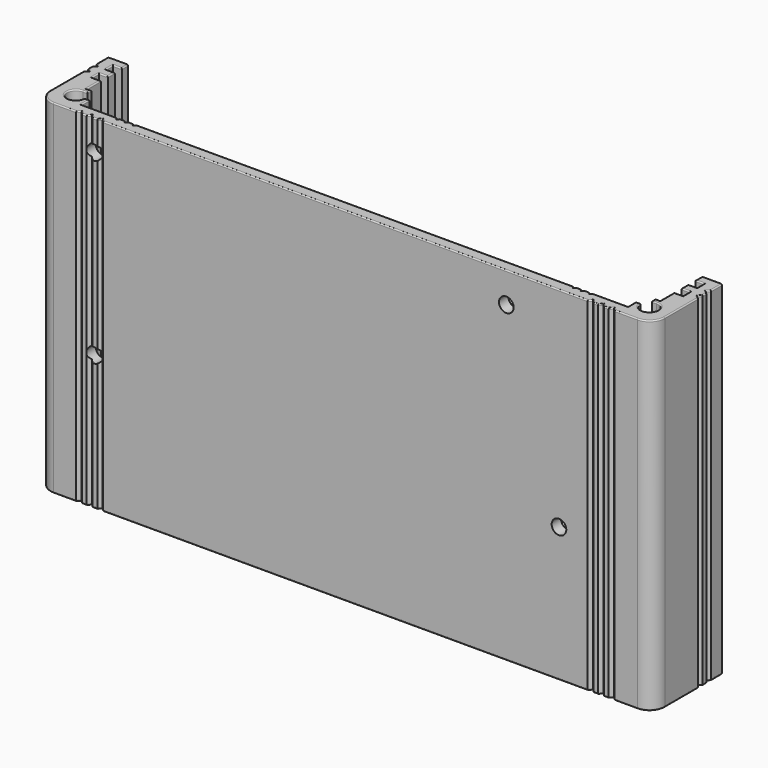
from build123d import *

# Parameters (mm, degrees)
F1_DEPTH     = 58.7
F2_R         = 0.2
F3_R         = 0.2
F4_T1_DEPTH  = 58.7
F4_T4_ANGLE  = 90
F4_T6_ANGLE  = 90
F4_T8_ANGLE  = 90
F4_T10_ANGLE = 90
F4_T12_ANGLE = 90
F4_T14_ANGLE = 90
F4_T16_ANGLE = 90
F4_T18_ANGLE = 90
F5_T1_DEPTH  = 58.7
F5_T4_ANGLE  = 90
F5_T6_ANGLE  = 90
F5_T8_ANGLE  = 90
F5_T10_ANGLE = 90
F6_R         = 1.25
F7_DEPTH     = 2


# Not quite as in the source:
# - a fillet or chamfer that OpenCascade refuses, or shapes differently, is made with other operations: its cross-section is extruded or revolved along the edge and cut away or added


with BuildPart() as f1:
    # F0 (on Top) → F1 (new body)
    with BuildSketch(Plane.XY):
        with BuildLine():
            Line((-52.5, -5.3), (-52.5, -15))
            Line((-52.5, -15), (-46, -15))
            Line((-46, -15), (-45.5, -14.5))
            Line((-45.5, -14.5), (-45, -15))
            Line((-45, -15), (-44.2, -15))
            Line((-44.2, -15), (-43.7, -14.5))
            Line((-43.7, -14.5), (-43.2, -15))
            Line((-43.2, -15), (-42.4, -15))
            Line((-42.4, -15), (-41.9, -14.5))
            Line((-41.9, -14.5), (-41.4, -15))
            Line((-41.4, -15), (0, -15))
            Line((0, -15), (41.4, -15))
            Line((41.4, -15), (41.9, -14.5))
            Line((41.9, -14.5), (42.4, -15))
            Line((42.4, -15), (43.2, -15))
            Line((43.2, -15), (43.7, -14.5))
            Line((43.7, -14.5), (44.2, -15))
            Line((44.2, -15), (45, -15))
            Line((45, -15), (45.5, -14.5))
            Line((45.5, -14.5), (46, -15))
            Line((46, -15), (52.5, -15))
            Line((52.5, -15), (52.5, -5.3))
            Line((52.5, -5.3), (52, -4.8))
            Line((52, -4.8), (52.5, -4.3))
            Line((52.5, -4.3), (52.5, -3.5))
            Line((52.5, -3.5), (52, -3))
            Line((52, -3), (52.5, -2.5))
            Line((52.5, -2.5), (52.5, 0))
            Line((52.5, 0), (49, 0))
            Line((49, 0), (49, -1.5))
            Line((49, -1.5), (50.5, -1.5))
            Line((50.5, -1.5), (50.5, -3))
            Line((50.5, -3), (49, -3))
            Line((49, -3), (49, -4.5))
            Line((49, -4.5), (50.5, -4.5))
            Line((50.5, -4.5), (50.5, -6))
            Line((50.5, -6), (49, -6))
            Line((49, -6), (49, -9))
            Line((49, -9), (48.2, -9))
            Line((48.2, -9), (48.2, -9.8))
            Line((48.2, -9.8), (49, -9.8))
            ThreePointArc((49, -9.8), (50.0606601718, -12.3606601718), (47.5, -11.3))
            Line((47.5, -11.3), (46.7, -11.3))
            Line((46.7, -11.3), (46.7, -13))
            Line((46.7, -13), (40.7, -13))
            Line((40.7, -13), (40.4, -13.3))
            Line((40.4, -13.3), (40.1, -13))
            Line((40.1, -13), (39.3, -13))
            Line((39.3, -13), (39, -13.3))
            Line((39, -13.3), (38.7, -13))
            Line((38.7, -13), (37.9, -13))
            Line((37.9, -13), (37.6, -13.3))
            Line((37.6, -13.3), (37.3, -13))
            Line((37.3, -13), (0, -13))
            Line((0, -13), (-37.3, -13))
            Line((-37.3, -13), (-37.6, -13.3))
            Line((-37.6, -13.3), (-37.9, -13))
            Line((-37.9, -13), (-38.7, -13))
            Line((-38.7, -13), (-39, -13.3))
            Line((-39, -13.3), (-39.3, -13))
            Line((-39.3, -13), (-40.1, -13))
            Line((-40.1, -13), (-40.4, -13.3))
            Line((-40.4, -13.3), (-40.7, -13))
            Line((-40.7, -13), (-46.7, -13))
            Line((-46.7, -13), (-46.7, -11.3))
            Line((-46.7, -11.3), (-47.5, -11.3))
            ThreePointArc((-47.5, -11.3), (-50.0606601718, -12.3606601718), (-49, -9.8))
            Line((-49, -9.8), (-48.2, -9.8))
            Line((-48.2, -9.8), (-48.2, -9))
            Line((-48.2, -9), (-49, -9))
            Line((-49, -9), (-49, -6))
            Line((-49, -6), (-50.5, -6))
            Line((-50.5, -6), (-50.5, -4.5))
            Line((-50.5, -4.5), (-49, -4.5))
            Line((-49, -4.5), (-49, -3))
            Line((-49, -3), (-50.5, -3))
            Line((-50.5, -3), (-50.5, -1.5))
            Line((-50.5, -1.5), (-49, -1.5))
            Line((-49, -1.5), (-49, 0))
            Line((-49, 0), (-52.5, 0))
            Line((-52.5, 0), (-52.5, -2.5))
            Line((-52.5, -2.5), (-52, -3))
            Line((-52, -3), (-52.5, -3.5))
            Line((-52.5, -3.5), (-52.5, -4.3))
            Line((-52.5, -4.3), (-52, -4.8))
            Line((-52, -4.8), (-52.5, -5.3))
        make_face()
    extrude(amount=F1_DEPTH)

    # F2
    f2_edges = [f1.edges().sort_by_distance(p)[0] for p in [
        (-52.5, -10.15, 58.7),
        (-49.25, -15, 58.7),
        (-45.75, -14.75, 58.7),
        (-45.25, -14.75, 58.7),
        (-44.6, -15, 58.7),
        (-43.95, -14.75, 58.7),
        (-43.45, -14.75, 58.7),
        (-42.8, -15, 58.7),
        (-42.15, -14.75, 58.7),
        (-41.65, -14.75, 58.7),
        (0, -15, 58.7),
        (41.65, -14.75, 58.7),
        (42.15, -14.75, 58.7),
        (42.8, -15, 58.7),
        (43.45, -14.75, 58.7),
        (43.95, -14.75, 58.7),
        (44.6, -15, 58.7),
        (45.25, -14.75, 58.7),
        (45.75, -14.75, 58.7),
        (49.25, -15, 58.7),
        (52.5, -10.15, 58.7),
        (52.25, -5.05, 58.7),
        (52.25, -4.55, 58.7),
        (52.5, -3.9, 58.7),
        (52.25, -3.25, 58.7),
        (52.25, -2.75, 58.7),
        (52.5, -1.25, 58.7),
        (50.75, 0, 58.7),
        (49, -0.75, 58.7),
        (49.75, -1.5, 58.7),
        (50.5, -2.25, 58.7),
        (49.75, -3, 58.7),
        (49, -3.75, 58.7),
        (49.75, -4.5, 58.7),
        (50.5, -5.25, 58.7),
        (49.75, -6, 58.7),
        (49, -7.5, 58.7),
        (48.6, -9, 58.7),
        (48.2, -9.4, 58.7),
        (48.6, -9.8, 58.7),
        (50.06066, -12.36066, 58.7),
        (47.1, -11.3, 58.7),
        (46.7, -12.15, 58.7),
        (43.7, -13, 58.7),
        (40.55, -13.15, 58.7),
        (40.25, -13.15, 58.7),
        (39.7, -13, 58.7),
        (39.15, -13.15, 58.7),
        (38.85, -13.15, 58.7),
        (38.3, -13, 58.7),
        (37.75, -13.15, 58.7),
        (37.45, -13.15, 58.7),
        (0, -13, 58.7),
        (-37.45, -13.15, 58.7),
        (-37.75, -13.15, 58.7),
        (-38.3, -13, 58.7),
        (-38.85, -13.15, 58.7),
        (-39.15, -13.15, 58.7),
        (-39.7, -13, 58.7),
        (-40.25, -13.15, 58.7),
        (-40.55, -13.15, 58.7),
        (-43.7, -13, 58.7),
        (-46.7, -12.15, 58.7),
        (-47.1, -11.3, 58.7),
        (-50.06066, -12.36066, 58.7),
        (-48.6, -9.8, 58.7),
        (-48.2, -9.4, 58.7),
        (-48.6, -9, 58.7),
        (-49, -7.5, 58.7),
        (-49.75, -6, 58.7),
        (-50.5, -5.25, 58.7),
        (-49.75, -4.5, 58.7),
        (-49, -3.75, 58.7),
        (-49.75, -3, 58.7),
        (-50.5, -2.25, 58.7),
        (-49.75, -1.5, 58.7),
        (-49, -0.75, 58.7),
        (-50.75, 0, 58.7),
        (-52.5, -1.25, 58.7),
        (-52.25, -2.75, 58.7),
        (-52.25, -3.25, 58.7),
        (-52.5, -3.9, 58.7),
        (-52.25, -4.55, 58.7),
        (-52.25, -5.05, 58.7),
    ]]
    fillet(f2_edges, radius=F2_R)

    # F3
    f3_edges = [f1.edges().sort_by_distance(p)[0] for p in [
        (-52.5, -10.15, 0),
        (-49.25, -15, 0),
        (-45.75, -14.75, 0),
        (-45.25, -14.75, 0),
        (-44.6, -15, 0),
        (-43.95, -14.75, 0),
        (-43.45, -14.75, 0),
        (-42.8, -15, 0),
        (-42.15, -14.75, 0),
        (-41.65, -14.75, 0),
        (0, -15, 0),
        (41.65, -14.75, 0),
        (42.15, -14.75, 0),
        (42.8, -15, 0),
        (43.45, -14.75, 0),
        (43.95, -14.75, 0),
        (44.6, -15, 0),
        (45.25, -14.75, 0),
        (45.75, -14.75, 0),
        (49.25, -15, 0),
        (52.5, -10.15, 0),
        (52.25, -5.05, 0),
        (52.25, -4.55, 0),
        (52.5, -3.9, 0),
        (52.25, -3.25, 0),
        (52.25, -2.75, 0),
        (52.5, -1.25, 0),
        (50.75, 0, 0),
        (49, -0.75, 0),
        (49.75, -1.5, 0),
        (50.5, -2.25, 0),
        (49.75, -3, 0),
        (49, -3.75, 0),
        (49.75, -4.5, 0),
        (50.5, -5.25, 0),
        (49.75, -6, 0),
        (49, -7.5, 0),
        (48.6, -9, 0),
        (48.2, -9.4, 0),
        (48.6, -9.8, 0),
        (50.06066, -12.36066, 0),
        (47.1, -11.3, 0),
        (46.7, -12.15, 0),
        (43.7, -13, 0),
        (40.55, -13.15, 0),
        (40.25, -13.15, 0),
        (39.7, -13, 0),
        (39.15, -13.15, 0),
        (38.85, -13.15, 0),
        (38.3, -13, 0),
        (37.75, -13.15, 0),
        (37.45, -13.15, 0),
        (0, -13, 0),
        (-37.45, -13.15, 0),
        (-37.75, -13.15, 0),
        (-38.3, -13, 0),
        (-38.85, -13.15, 0),
        (-39.15, -13.15, 0),
        (-39.7, -13, 0),
        (-40.25, -13.15, 0),
        (-40.55, -13.15, 0),
        (-43.7, -13, 0),
        (-46.7, -12.15, 0),
        (-47.1, -11.3, 0),
        (-50.06066, -12.36066, 0),
        (-48.6, -9.8, 0),
        (-48.2, -9.4, 0),
        (-48.6, -9, 0),
        (-49, -7.5, 0),
        (-49.75, -6, 0),
        (-50.5, -5.25, 0),
        (-49.75, -4.5, 0),
        (-49, -3.75, 0),
        (-49.75, -3, 0),
        (-50.5, -2.25, 0),
        (-49.75, -1.5, 0),
        (-49, -0.75, 0),
        (-50.75, 0, 0),
        (-52.5, -1.25, 0),
        (-52.25, -2.75, 0),
        (-52.25, -3.25, 0),
        (-52.5, -3.9, 0),
        (-52.25, -4.55, 0),
        (-52.25, -5.05, 0),
    ]]
    fillet(f3_edges, radius=F3_R)

    # F4: fillet of radius 0.3 on 4 edges, made by hand

    # F4_s2 → F4_t1 (cut)
    with BuildSketch(Plane.XY):
        with BuildLine():
            ThreePointArc((-52.5, -0.3), (-52.4121320344, -0.0878679656), (-52.2, 0))
            Line((-52.2, 0), (-52.5, 0))
            Line((-52.5, 0), (-52.5, -0.3))
        make_face()
        with BuildLine():
            ThreePointArc((-49.3, 0), (-49.0878679656, -0.0878679656), (-49, -0.3))
            Line((-49, -0.3), (-49, 0))
            Line((-49, 0), (-49.3, 0))
        make_face()
        with BuildLine():
            ThreePointArc((49.3, 0), (49.0878679656, -0.0878679656), (49, -0.3))
            Line((49, -0.3), (49, 0))
            Line((49, 0), (49.3, 0))
        make_face()
        with BuildLine():
            ThreePointArc((52.5, -0.3), (52.4121320344, -0.0878679656), (52.2, 0))
            Line((52.2, 0), (52.5, 0))
            Line((52.5, 0), (52.5, -0.3))
        make_face()
    extrude(amount=F4_T1_DEPTH, mode=Mode.SUBTRACT)

    # F4_s3 → F4_t4 (revolve, cut)
    with BuildSketch(Plane.YZ.offset(52.2)):
        with BuildLine():
            ThreePointArc((-0.2, 0), (-0.0585786438, 0.0585786438), (0, 0.2))
            Line((0, 0.2), (0, 0))
            Line((0, 0), (-0.2, 0))
        make_face()
    revolve(axis=Axis((52.2, -0.3, 0), (0, 0, -1)), revolution_arc=F4_T4_ANGLE, mode=Mode.SUBTRACT)

    # F4_s5 → F4_t6 (revolve, cut)
    with BuildSketch(Plane.XZ.offset(0.3)):
        with BuildLine():
            ThreePointArc((52.3, 58.7), (52.4414213562, 58.6414213562), (52.5, 58.5))
            Line((52.5, 58.5), (52.5, 58.7))
            Line((52.5, 58.7), (52.3, 58.7))
        make_face()
    revolve(axis=Axis((52.2, -0.3, 58.7), (0, 0, 1)), revolution_arc=F4_T6_ANGLE, mode=Mode.SUBTRACT)

    # F4_s7 → F4_t8 (revolve, cut)
    with BuildSketch(Plane.XZ.offset(0.3)):
        with BuildLine():
            ThreePointArc((49.2, 0), (49.0585786438, 0.0585786438), (49, 0.2))
            Line((49, 0.2), (49, 0))
            Line((49, 0), (49.2, 0))
        make_face()
    revolve(axis=Axis((49.3, -0.3, 0), (0, 0, -1)), revolution_arc=F4_T8_ANGLE, mode=Mode.SUBTRACT)

    # F4_s9 → F4_t10 (revolve, cut)
    with BuildSketch(Plane.YZ.offset(49.3)):
        with BuildLine():
            ThreePointArc((-0.2, 58.7), (-0.0585786438, 58.6414213562), (0, 58.5))
            Line((0, 58.5), (0, 58.7))
            Line((0, 58.7), (-0.2, 58.7))
        make_face()
    revolve(axis=Axis((49.3, -0.3, 58.7), (0, 0, 1)), revolution_arc=F4_T10_ANGLE, mode=Mode.SUBTRACT)

    # F4_s11 → F4_t12 (revolve, cut)
    with BuildSketch(Plane.YZ.offset(-49.3)):
        with BuildLine():
            ThreePointArc((-0.2, 0), (-0.0585786438, 0.0585786438), (0, 0.2))
            Line((0, 0.2), (0, 0))
            Line((0, 0), (-0.2, 0))
        make_face()
    revolve(axis=Axis((-49.3, -0.3, 0), (0, 0, -1)), revolution_arc=F4_T12_ANGLE, mode=Mode.SUBTRACT)

    # F4_s13 → F4_t14 (revolve, cut)
    with BuildSketch(Plane.XZ.offset(0.3)):
        with BuildLine():
            ThreePointArc((-49.2, 58.7), (-49.0585786438, 58.6414213562), (-49, 58.5))
            Line((-49, 58.5), (-49, 58.7))
            Line((-49, 58.7), (-49.2, 58.7))
        make_face()
    revolve(axis=Axis((-49.3, -0.3, 58.7), (0, 0, 1)), revolution_arc=F4_T14_ANGLE, mode=Mode.SUBTRACT)

    # F4_s15 → F4_t16 (revolve, cut)
    with BuildSketch(Plane.XZ.offset(0.3)):
        with BuildLine():
            ThreePointArc((-52.3, 0), (-52.4414213562, 0.0585786438), (-52.5, 0.2))
            Line((-52.5, 0.2), (-52.5, 0))
            Line((-52.5, 0), (-52.3, 0))
        make_face()
    revolve(axis=Axis((-52.2, -0.3, 0), (0, 0, -1)), revolution_arc=F4_T16_ANGLE, mode=Mode.SUBTRACT)

    # F4_s17 → F4_t18 (revolve, cut)
    with BuildSketch(Plane.YZ.offset(-52.2)):
        with BuildLine():
            ThreePointArc((-0.2, 58.7), (-0.0585786438, 58.6414213562), (0, 58.5))
            Line((0, 58.5), (0, 58.7))
            Line((0, 58.7), (-0.2, 58.7))
        make_face()
    revolve(axis=Axis((-52.2, -0.3, 58.7), (0, 0, 1)), revolution_arc=F4_T18_ANGLE, mode=Mode.SUBTRACT)

    # F5: fillet of radius 2.6 on 2 edges, made by hand

    # F5_s2 → F5_t1 (cut)
    with BuildSketch(Plane.XY):
        with BuildLine():
            ThreePointArc((-52.5, -12.4), (-51.7384776311, -14.2384776311), (-49.9, -15))
            Line((-49.9, -15), (-52.5, -15))
            Line((-52.5, -15), (-52.5, -12.4))
        make_face()
        with BuildLine():
            ThreePointArc((52.5, -12.4), (51.7384776311, -14.2384776311), (49.9, -15))
            Line((49.9, -15), (52.5, -15))
            Line((52.5, -15), (52.5, -12.4))
        make_face()
    extrude(amount=F5_T1_DEPTH, mode=Mode.SUBTRACT)

    # F5_s3 → F5_t4 (revolve, cut)
    with BuildSketch(Plane.XZ.offset(12.4)):
        with BuildLine():
            ThreePointArc((52.3, 0), (52.4414213562, 0.0585786438), (52.5, 0.2))
            Line((52.5, 0.2), (52.5, 0))
            Line((52.5, 0), (52.3, 0))
        make_face()
    revolve(axis=Axis((49.9, -12.4, 0), (0, 0, -1)), revolution_arc=F5_T4_ANGLE, mode=Mode.SUBTRACT)

    # F5_s5 → F5_t6 (revolve, cut)
    with BuildSketch(Plane.YZ.offset(49.9)):
        with BuildLine():
            ThreePointArc((-14.8, 58.7), (-14.9414213562, 58.6414213562), (-15, 58.5))
            Line((-15, 58.5), (-15, 58.7))
            Line((-15, 58.7), (-14.8, 58.7))
        make_face()
    revolve(axis=Axis((49.9, -12.4, 58.7), (0, 0, 1)), revolution_arc=F5_T6_ANGLE, mode=Mode.SUBTRACT)

    # F5_s7 → F5_t8 (revolve, cut)
    with BuildSketch(Plane.YZ.offset(-49.9)):
        with BuildLine():
            ThreePointArc((-14.8, 0), (-14.9414213562, 0.0585786438), (-15, 0.2))
            Line((-15, 0.2), (-15, 0))
            Line((-15, 0), (-14.8, 0))
        make_face()
    revolve(axis=Axis((-49.9, -12.4, 0), (0, 0, -1)), revolution_arc=F5_T8_ANGLE, mode=Mode.SUBTRACT)

    # F5_s9 → F5_t10 (revolve, cut)
    with BuildSketch(Plane.XZ.offset(12.4)):
        with BuildLine():
            ThreePointArc((-52.3, 58.7), (-52.4414213562, 58.6414213562), (-52.5, 58.5))
            Line((-52.5, 58.5), (-52.5, 58.7))
            Line((-52.5, 58.7), (-52.3, 58.7))
        make_face()
    revolve(axis=Axis((-49.9, -12.4, 58.7), (0, 0, 1)), revolution_arc=F5_T10_ANGLE, mode=Mode.SUBTRACT)

    # F6 (on face) → F7 (cut, through all)
    with BuildSketch(Plane(origin=(0, -13, 0), x_dir=(-1, 0, 0), z_dir=(0, 1, 0))):
        with Locations((-27.5, 53.5)):
            Circle(F6_R)
        with Locations((-36.5, 23)):
            Circle(F6_R)
        with Locations((43, 53.5)):
            Circle(F6_R)
        with Locations((43, 23)):
            Circle(F6_R)
    extrude(amount=-F7_DEPTH, mode=Mode.SUBTRACT)


solid = f1.part
